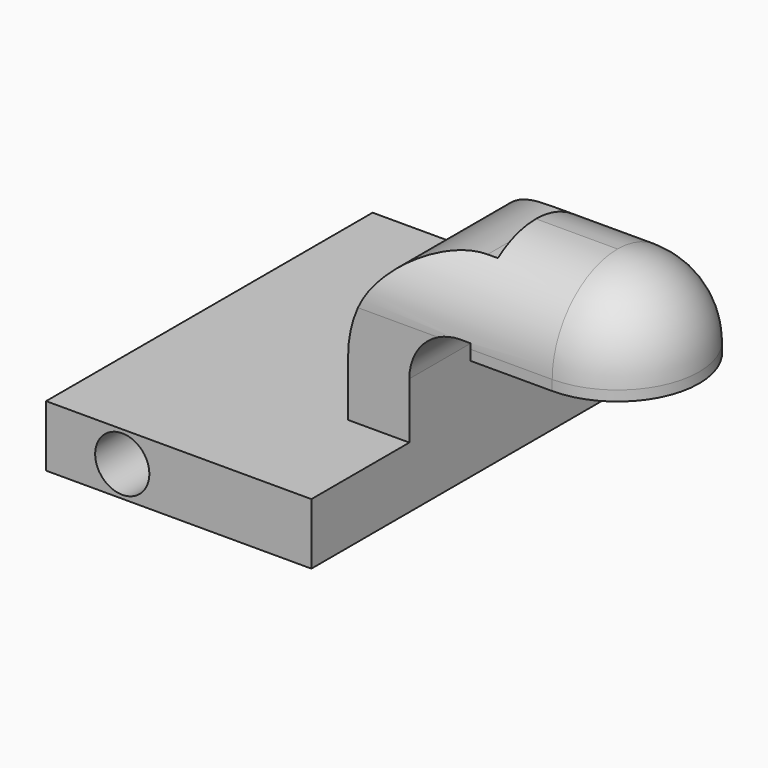
from build123d import *

# Parameters (mm, degrees)
F0_R        = 8.4292164968
F1_DEPTH    = 63.5
F0_W        = 25.4
F0_H        = 19.05
F2_DEPTH    = 25.4
F0_H_2      = 4.7498
F0_H_3      = 4.7752
F4_DEPTH    = 25.4
F5_DEPTH    = 25.4
F6_T1_DEPTH = 88.9
F6_T4_ANGLE = 180
F7_T        = 2.54
F7_T3_DEPTH = 24.13
F7_T5_DEPTH = 55.88
F7_T7_DEPTH = 55.7790871697
F7_T9_DEPTH = 34.6589952471


# Not quite as in the source:
# - a fillet or chamfer that OpenCascade refuses, or shapes differently, is made with other operations: its cross-section is extruded or revolved along the edge and cut away or added
# - a feature of the source that left no trace in its solid (it failed there, or was rolled back) is left out
# - a shell that OpenCascade refuses in one call is made with other operations: the cavity is built on its own and cut out


with BuildPart() as f1:
    # F0 (on Front) → F1 (new body, symmetric)
    with BuildSketch(Plane.XZ):
        Polygon((-41.275, -9.525), (41.275, -9.525), (41.275, 9.525), (22.225, 9.525), (-41.275, 9.525), align=None)
        with Locations((-17.5714660436, 0)):
            Circle(F0_R, mode=Mode.SUBTRACT)
    extrude(amount=F1_DEPTH, both=True)

    # F0 (on Front) → F2 (join, symmetric)
    with BuildSketch(Plane.XZ):
        with BuildLine():
            Line((60.325, 61.9252), (57.15, 61.9252))
            ThreePointArc((57.15, 61.9252), (32.4542956671, 51.6959043329), (22.225, 27.0002))
            Line((22.225, 27.0002), (22.225, 9.525))
            Line((22.225, 9.525), (41.275, 9.525))
            Line((41.275, 9.525), (41.275, 27.0002))
            ThreePointArc((41.275, 27.0002), (45.9246798487, 38.2255201513), (57.15, 42.8752))
            Line((57.15, 42.8752), (60.325, 42.8752))
            Line((60.325, 42.8752), (60.325, 61.9252))
        make_face()
        with Locations((73.025, 52.4002)):
            Rectangle(F0_W, F0_H)
    extrude(amount=F2_DEPTH, both=True)

    # F0 (on Front) → F3 (revolve)
    with BuildSketch(Plane.XZ):
        Polygon((85.725, 66.675), (85.725, 61.9252), (85.725, 42.8752), (85.725, 38.1), (111.125, 38.1), (111.125, 66.675), align=None)
    revolve(axis=Axis((85.725, 0, 52.3875), (0, 0, 1)))

    # F0 (on Front) → F4 (join)
    with BuildSketch(Plane.XZ):
        with Locations((73.025, 64.3001)):
            Rectangle(F0_W, F0_H_2)
        with Locations((73.025, 40.4876)):
            Rectangle(F0_W, F0_H_3)
    extrude(amount=F4_DEPTH)

    # F0 (on Front) → F5 (join)
    with BuildSketch(Plane.XZ):
        with Locations((73.025, 40.4876)):
            Rectangle(F0_W, F0_H_3)
        with Locations((73.025, 64.3001)):
            Rectangle(F0_W, F0_H_2)
    extrude(amount=-F5_DEPTH)

    # F6: fillet of radius 25.4 on 3 edges, made by hand

    # F6_s2 → F6_t1 (cut)
    with BuildSketch(Plane.YZ.offset(-3.175)):
        with BuildLine():
            ThreePointArc((-25.4, 41.275), (-17.9605122421, 59.2355122421), (0, 66.675))
            Line((0, 66.675), (-25.4, 66.675))
            Line((-25.4, 66.675), (-25.4, 41.275))
        make_face()
        with BuildLine():
            ThreePointArc((0, 66.675), (17.9605122421, 59.2355122421), (25.4, 41.275))
            Line((25.4, 41.275), (25.4, 66.675))
            Line((25.4, 66.675), (0, 66.675))
        make_face()
    extrude(amount=F6_T1_DEPTH, mode=Mode.SUBTRACT)

    # F6_s3 → F6_t4 (revolve, cut)
    with BuildSketch(Plane.YZ.offset(85.725)):
        with BuildLine():
            ThreePointArc((0, 66.675), (17.9605122421, 59.2355122421), (25.4, 41.275))
            Line((25.4, 41.275), (25.4, 66.675))
            Line((25.4, 66.675), (0, 66.675))
        make_face()
    revolve(axis=Axis((85.725, 0, 66.675), (0, 0, -1)), revolution_arc=F6_T4_ANGLE, mode=Mode.SUBTRACT)

    # F7: shell of thickness 2.54, made by hand


with BuildPart() as f7_core1:
    # F7_t2: copy of F1
    add(f1.part)

    # the walls: a layer under each face that stays
    f7_faces = [f7_core1.faces().sort_by_distance(p)[0] for p in [
        (0, 0, -9.525),
        (0, 63.5, 0),
        (41.275, 0, 8.7376),
        (0, -63.5, 0),
        (-41.275, 0, 0),
        (0, 0, 9.525),
        (-26.0006825404, 0, 0),
        (36.214543408, 25.4, 25.4),
        (45.9246798487, 0, 38.2255201513),
        (36.214543408, -25.4, 25.4),
        (22.225, 0, 18.2626),
        (55.5002346295, 17.9605122421, 59.2355122421),
        (32.4542956671, 0, 51.6959043329),
        (55.5002346295, -17.9605122421, 59.2355122421),
        (58.7375, 0, 42.8752),
        (60.325, 0, 64.3001),
        (58.7375, 0, 61.9252),
        (60.325, 0, 40.4876),
        (73.025, 25.4, 39.6875),
        (103.6855122422, -1e-10, 59.2355122421),
        (73.025, -25.4, 39.6875),
        (111.125, 0, 39.6875),
    ]]
    thicken(f7_faces, amount=-F7_T, mode=Mode.SUBTRACT)

    # F7_s4 → F7_t3 (cut)
    with BuildSketch(Plane.YZ.offset(19.685)):
        Polygon((25.4254, 9.5504), (25.4, 6.985), (22.86, 6.985), (22.86, 9.525), align=None)
        Polygon((-25.4254, 9.5504), (-25.4, 6.985), (-22.86, 6.985), (-22.86, 9.525), align=None)
    extrude(amount=F7_T3_DEPTH, mode=Mode.SUBTRACT)

    # F7_s6 → F7_t5 (cut)
    with BuildSketch(Plane.XZ.offset(-27.94)):
        Polygon((22.1996, 9.5504), (22.225, 6.985), (24.765, 6.985), (24.765, 9.525), align=None)
    extrude(amount=F7_T5_DEPTH, mode=Mode.SUBTRACT)

    # F7_s8 → F7_t7 (cut)
    with BuildSketch(Plane.XZ.offset(-27.8895435848)):
        Polygon((60.2996, 42.8498), (60.325, 45.4152), (62.865, 45.4152), (62.865, 42.8752), align=None)
    extrude(amount=F7_T7_DEPTH, mode=Mode.SUBTRACT)

    # F7_s10 → F7_t9 (cut)
    with BuildSketch(Plane.XZ.offset(-17.3294976236)):
        Polygon((60.2996, 61.9506), (62.865, 61.9252), (62.865, 59.3852), (60.325, 59.3852), align=None)
    extrude(amount=F7_T9_DEPTH, mode=Mode.SUBTRACT)


with BuildPart() as f1_1:
    add(f1.part)

    # what is left inside the walls is the cavity
    f7_cavity = [f7_core1.part.solids().sort_by_distance(p)[0] for p in [
        (-28.566083, -20.32, 0),
        (14.810641, 20.32, -6.9596),
    ]]
    add(f7_cavity, mode=Mode.SUBTRACT)


solid = f1_1.part
